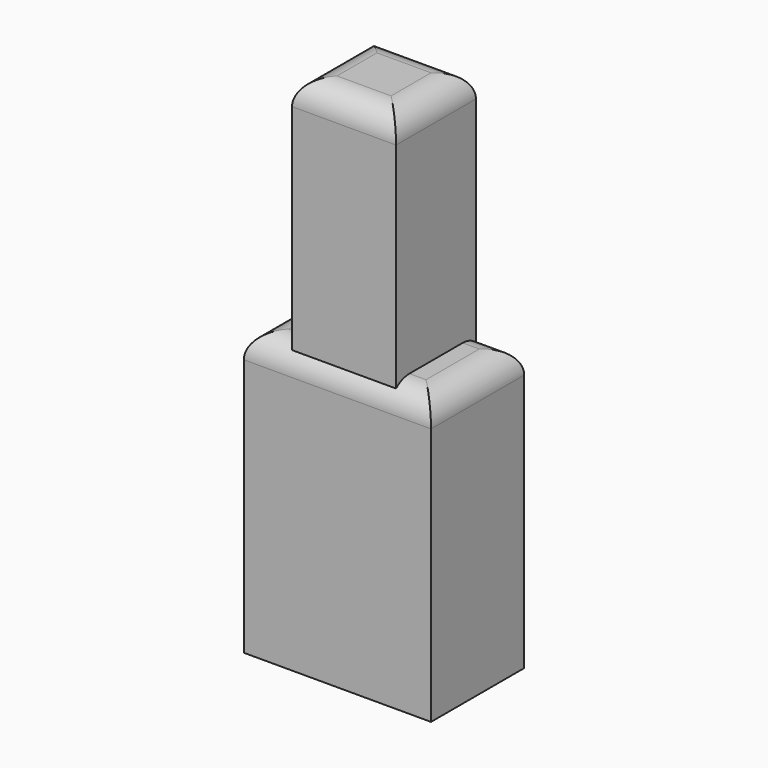
from build123d import *

# Parameters (mm, degrees)
F0_W         = 12.5
F0_H         = 12
F0_W_2       = 10.5
F0_H_2       = 10
F1_DEPTH     = 62
F0_W_3       = 22.5
F0_H_3       = 14
F0_W_4       = 4
F2_DEPTH     = 34
F3_DEPTH     = 60
F4_DEPTH     = 32
F5_R         = 3
F6_T1_DEPTH  = 29
F6_T6_DEPTH  = 37.5
F6_T11_DEPTH = 37.5
F6_T16_DEPTH = 37.5
F6_T21_DEPTH = 37.5
F6_T26_DEPTH = 37.5
F6_T31_DEPTH = 37.5


# Not quite as in the source:
# - a fillet or chamfer that OpenCascade refuses, or shapes differently, is made with other operations: its cross-section is extruded or revolved along the edge and cut away or added


with BuildPart() as f1:
    # F0 (on Top) → F1 (new body)
    with BuildSketch(Plane.XY):
        Rectangle(F0_W, F0_H)
        Rectangle(F0_W_2, F0_H_2, mode=Mode.SUBTRACT)
        Rectangle(F0_W_2, F0_H_2)
    extrude(amount=F1_DEPTH)

    # F0 (on Top) → F2 (join)
    with BuildSketch(Plane.XY):
        Rectangle(F0_W_3, F0_H_3)
        Polygon((-10.25, -6), (-10.25, 6), (-6.25, 6), (6.25, 6), (10.25, 6), (10.25, -6), (6.25, -6), (-6.25, -6), align=None, mode=Mode.SUBTRACT)
        with Locations((-8.25, 0)):
            Rectangle(F0_W_4, F0_H)
        with Locations((8.25, 0)):
            Rectangle(F0_W_4, F0_H)
    extrude(amount=F2_DEPTH)

    # F0 (on Top) → F3 (cut)
    with BuildSketch(Plane.XY):
        Rectangle(F0_W_2, F0_H_2)
    extrude(amount=F3_DEPTH, mode=Mode.SUBTRACT)

    # F0 (on Top) → F4 (cut)
    with BuildSketch(Plane.XY):
        Rectangle(F0_W, F0_H)
        Rectangle(F0_W_2, F0_H_2, mode=Mode.SUBTRACT)
        with Locations((-8.25, 0)):
            Rectangle(F0_W_4, F0_H)
        with Locations((8.25, 0)):
            Rectangle(F0_W_4, F0_H)
    extrude(amount=F4_DEPTH, mode=Mode.SUBTRACT)

    # F5
    f5_edges = [f1.edges().sort_by_distance(p)[0] for p in [
        (0, 6, 62),
        (-6.25, 0, 62),
        (0, -6, 62),
        (6.25, 0, 62),
    ]]
    fillet(f5_edges, radius=F5_R)

    # F6: fillet of radius 3 on 4 edges, made by hand

    # F6_s2 → F6_t1 (cut)
    with BuildSketch(Plane.XZ.offset(-14.5)):
        with BuildLine():
            ThreePointArc((-8.25, 34), (-10.3713203436, 33.1213203436), (-11.25, 31))
            Line((-11.25, 31), (-11.25, 34))
            Line((-11.25, 34), (-8.25, 34))
        make_face()
        with BuildLine():
            ThreePointArc((8.25, 34), (10.3713203436, 33.1213203436), (11.25, 31))
            Line((11.25, 31), (11.25, 34))
            Line((11.25, 34), (8.25, 34))
        make_face()
    extrude(amount=F6_T1_DEPTH, mode=Mode.SUBTRACT)


with BuildPart() as f6_tool4:
    # F6_s5 → F6_t6 (new body)
    with BuildSketch(Plane.YZ.offset(-18.75)):
        with BuildLine():
            ThreePointArc((-4, 34), (-6.1213203436, 33.1213203436), (-7, 31))
            Line((-7, 31), (-7, 34))
            Line((-7, 34), (-4, 34))
        make_face()
    extrude(amount=F6_T6_DEPTH)

    split(bisect_by=Plane.YZ.offset(-6.25), keep=Keep.BOTTOM)


with BuildPart() as f1_1:
    add(f1.part)

    # F6_t3: cut F6_tool4
    add(f6_tool4.part, mode=Mode.SUBTRACT)


with BuildPart() as f6_tool9:
    # F6_s10 → F6_t11 (new body)
    with BuildSketch(Plane.YZ.offset(-18.75)):
        with BuildLine():
            ThreePointArc((-4, 34), (-6.1213203436, 33.1213203436), (-7, 31))
            Line((-7, 31), (-7, 34))
            Line((-7, 34), (-4, 34))
        make_face()
    extrude(amount=F6_T11_DEPTH)

    split(bisect_by=Plane.XZ.offset(6), keep=Keep.TOP)


with BuildPart() as f1_2:
    add(f1_1.part)

    # F6_t8: cut F6_tool9
    add(f6_tool9.part, mode=Mode.SUBTRACT)


with BuildPart() as f6_tool14:
    # F6_s15 → F6_t16 (new body)
    with BuildSketch(Plane.YZ.offset(-18.75)):
        with BuildLine():
            ThreePointArc((-4, 34), (-6.1213203436, 33.1213203436), (-7, 31))
            Line((-7, 31), (-7, 34))
            Line((-7, 34), (-4, 34))
        make_face()
    extrude(amount=F6_T16_DEPTH)

    split(bisect_by=Plane.YZ.offset(6.25), keep=Keep.TOP)


with BuildPart() as f1_3:
    add(f1_2.part)

    # F6_t13: cut F6_tool14
    add(f6_tool14.part, mode=Mode.SUBTRACT)


with BuildPart() as f6_tool19:
    # F6_s20 → F6_t21 (new body)
    with BuildSketch(Plane.YZ.offset(18.75)):
        with BuildLine():
            ThreePointArc((4, 34), (6.1213203436, 33.1213203436), (7, 31))
            Line((7, 31), (7, 34))
            Line((7, 34), (4, 34))
        make_face()
    extrude(amount=-F6_T21_DEPTH)

    split(bisect_by=Plane.YZ.offset(6.25), keep=Keep.TOP)


with BuildPart() as f1_4:
    add(f1_3.part)

    # F6_t18: cut F6_tool19
    add(f6_tool19.part, mode=Mode.SUBTRACT)


with BuildPart() as f6_tool24:
    # F6_s25 → F6_t26 (new body)
    with BuildSketch(Plane.YZ.offset(18.75)):
        with BuildLine():
            ThreePointArc((4, 34), (6.1213203436, 33.1213203436), (7, 31))
            Line((7, 31), (7, 34))
            Line((7, 34), (4, 34))
        make_face()
    extrude(amount=-F6_T26_DEPTH)

    split(bisect_by=Plane.XZ.offset(-6), keep=Keep.BOTTOM)


with BuildPart() as f1_5:
    add(f1_4.part)

    # F6_t23: cut F6_tool24
    add(f6_tool24.part, mode=Mode.SUBTRACT)


with BuildPart() as f6_tool29:
    # F6_s30 → F6_t31 (new body)
    with BuildSketch(Plane.YZ.offset(18.75)):
        with BuildLine():
            ThreePointArc((4, 34), (6.1213203436, 33.1213203436), (7, 31))
            Line((7, 31), (7, 34))
            Line((7, 34), (4, 34))
        make_face()
    extrude(amount=-F6_T31_DEPTH)

    split(bisect_by=Plane.YZ.offset(-6.25), keep=Keep.BOTTOM)


with BuildPart() as f1_6:
    add(f1_5.part)

    # F6_t28: cut F6_tool29
    add(f6_tool29.part, mode=Mode.SUBTRACT)


solid = f1_6.part
